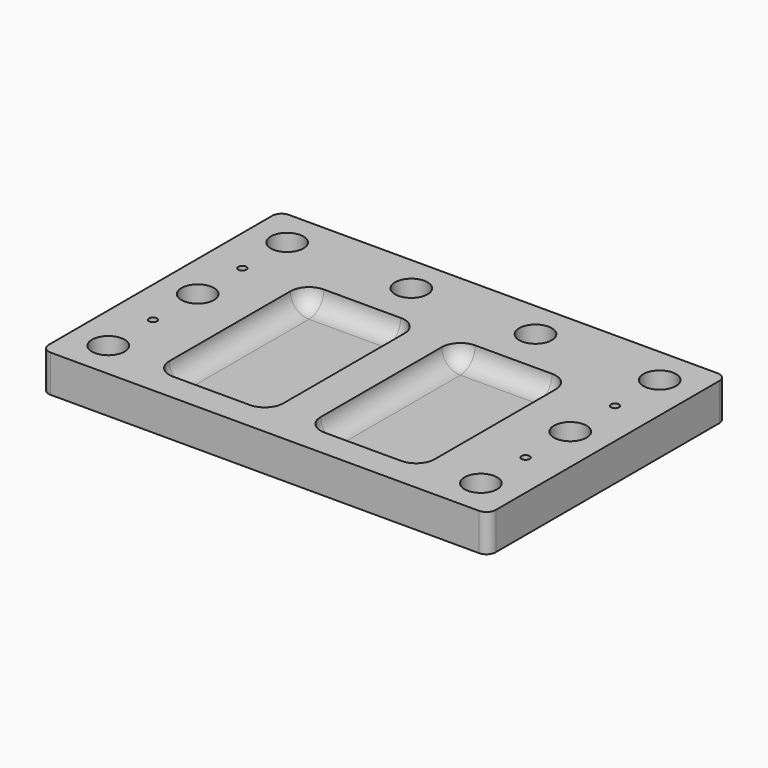
from build123d import *

# Parameters (mm, degrees)
F1_DEPTH = 12.7
F3_R     = 5.55625
F4_DEPTH = 12.701
F2_R     = 1.3890625
F5_DEPTH = 12.701
F7_DEPTH = 6.35
F8_R     = 6.34999
F9_R     = 6.34999


# Not quite as in the source:
# - a fillet or chamfer is up to 0.001 mm smaller than in the source, because OpenCascade refuses the exact size


with BuildPart() as f1:
    # F0 (on Top) → F1 (new body)
    with BuildSketch(Plane.XY):
        with BuildLine():
            Line((-73.025, -50.8), (73.025, -50.8))
            ThreePointArc((73.025, -50.8), (75.2700640303, -49.8700640303), (76.2, -47.625))
            Line((76.2, -47.625), (76.2, 47.625))
            ThreePointArc((76.2, 47.625), (75.2700640303, 49.8700640303), (73.025, 50.8))
            Line((73.025, 50.8), (-73.025, 50.8))
            ThreePointArc((-73.025, 50.8), (-75.2700640303, 49.8700640303), (-76.2, 47.625))
            Line((-76.2, 47.625), (-76.2, -47.625))
            ThreePointArc((-76.2, -47.625), (-75.2700640303, -49.8700640303), (-73.025, -50.8))
        make_face()
    extrude(amount=F1_DEPTH)

    # F3 (on face) → F4 (cut, through all)
    with BuildSketch(Plane.XY.offset(12.7)):
        with Locations((-63.5, 38.1)):
            Circle(F3_R)
        with Locations((63.5, 38.1)):
            Circle(F3_R)
        with Locations((63.5, -38.1)):
            Circle(F3_R)
        with Locations((-63.5, -38.1)):
            Circle(F3_R)
        with Locations((-63.5, 0)):
            Circle(F3_R)
        with Locations((63.5, 0)):
            Circle(F3_R)
        with Locations((-21.1666666667, 38.1)):
            Circle(F3_R)
        with Locations((21.1666666667, 38.1)):
            Circle(F3_R)
    extrude(amount=-F4_DEPTH, mode=Mode.SUBTRACT)

    # F2 (on face) → F5 (cut, through all)
    with BuildSketch(Plane.XY.offset(12.7)):
        with Locations((-63.5, -19.05)):
            Circle(F2_R)
        with Locations((63.5, 19.05)):
            Circle(F2_R)
        with Locations((63.5, -19.05)):
            Circle(F2_R)
        with Locations((-63.5, 19.05)):
            Circle(F2_R)
    extrude(amount=-F5_DEPTH, mode=Mode.SUBTRACT)

    # F6 (on face) → F7 (cut)
    with BuildSketch(Plane.XY.offset(12.7)):
        with BuildLine():
            ThreePointArc((-6.35, 16.66875), (-8.2098719395, 21.1588780605), (-12.7, 23.01875))
            Line((-12.7, 23.01875), (-38.89375, 23.01875))
            ThreePointArc((-38.89375, 23.01875), (-43.3838780605, 21.1588780605), (-45.24375, 16.66875))
            Line((-45.24375, 16.66875), (-45.24375, -34.925))
            ThreePointArc((-45.24375, -34.925), (-43.3838780605, -39.4151280605), (-38.89375, -41.275))
            Line((-38.89375, -41.275), (-12.7, -41.275))
            ThreePointArc((-12.7, -41.275), (-8.2098719395, -39.4151280605), (-6.35, -34.925))
            Line((-6.35, -34.925), (-6.35, 16.66875))
        make_face()
        with BuildLine():
            ThreePointArc((6.35, -34.925), (8.2098719395, -39.4151280605), (12.7, -41.275))
            Line((12.7, -41.275), (38.89375, -41.275))
            ThreePointArc((38.89375, -41.275), (43.3838780605, -39.4151280605), (45.24375, -34.925))
            Line((45.24375, -34.925), (45.24375, 16.66875))
            ThreePointArc((45.24375, 16.66875), (43.3838780605, 21.1588780605), (38.89375, 23.01875))
            Line((38.89375, 23.01875), (12.7, 23.01875))
            ThreePointArc((12.7, 23.01875), (8.2098719395, 21.1588780605), (6.35, 16.66875))
            Line((6.35, 16.66875), (6.35, -34.925))
        make_face()
    extrude(amount=-F7_DEPTH, mode=Mode.SUBTRACT)

    # F8 (radius 6.35 in the source; OpenCascade refuses exactly that, so slightly less here)
    f8_edges = [f1.edges().sort_by_distance(p)[0] for p in [
        (-25.796875, -41.275, 6.35),
        (-6.35, -9.128125, 6.35),
        (-8.209872, -39.415128, 6.35),
        (-45.24375, -9.128125, 6.35),
        (-43.383878, -39.415128, 6.35),
        (-43.383878, 21.158878, 6.35),
        (-25.796875, 23.01875, 6.35),
        (-8.209872, 21.158878, 6.35),
    ]]
    fillet(f8_edges, radius=F8_R)

    # F9 (radius 6.35 in the source; OpenCascade refuses exactly that, so slightly less here)
    f9_edges = [f1.edges().sort_by_distance(p)[0] for p in [
        (6.35, -9.128125, 6.35),
        (8.209872, 21.158878, 6.35),
        (25.796875, 23.01875, 6.35),
        (43.383878, 21.158878, 6.35),
        (45.24375, -9.128125, 6.35),
        (43.383878, -39.415128, 6.35),
        (25.796875, -41.275, 6.35),
        (8.209872, -39.415128, 6.35),
    ]]
    fillet(f9_edges, radius=F9_R)


solid = f1.part
